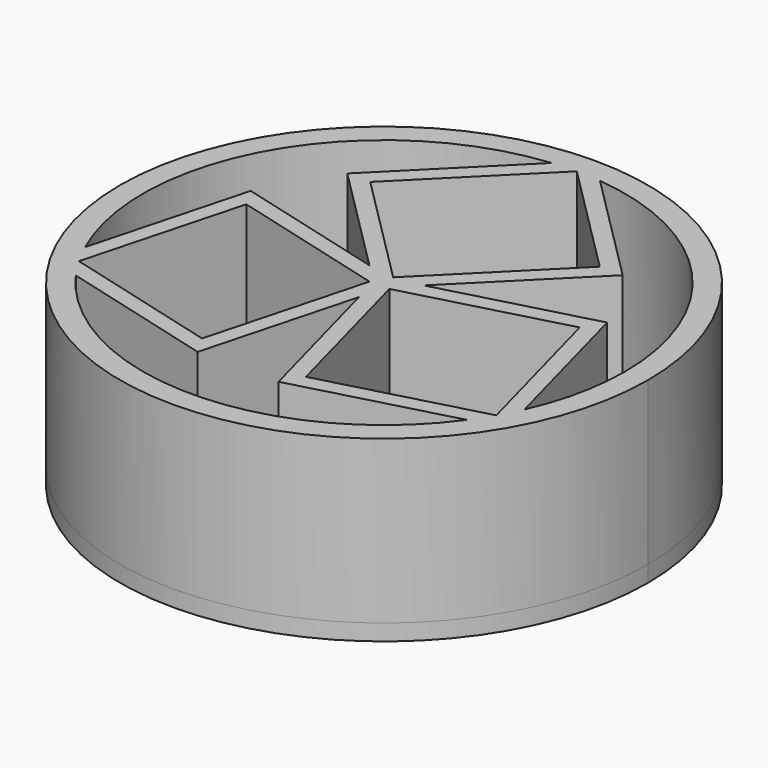
from build123d import *
from build123d import SkipClean  # not in build123d's __all__

# Parameters (mm, degrees)
F1_DEPTH = 1
F2_DEPTH = 10


with BuildPart() as f1:
    # F0 (on Top) → F1 (new body)
    with BuildSketch(Plane.XY):
        with BuildLine():
            Line((10.9787374798, 3.4593819318), (1.6730326075, 0.9659258263))
            Line((1.6730326075, 0.9659258263), (0.4482877361, -0.2588190451))
            Line((0.4482877361, -0.2588190451), (0, -1.9318516526))
            Line((0, -1.9318516526), (2.4934561055, -11.2375565249))
            Line((2.4934561055, -11.2375565249), (12.0504683321, -8.6767628167))
            ThreePointArc((12.0504683321, -8.6767628167), (12.4708698642, -8.0608563335), (12.8598211496, -7.4246212025))
            ThreePointArc((12.8598211496, -7.4246212025), (13.2163412932, -6.769661943), (13.5395311879, -6.0976302947))
            Line((13.5395311879, -6.0976302947), (10.9787374798, 3.4593819318))
        make_face()
        Polygon((10.2716306986, 2.2346370604), (12.8598211496, -7.4246212025), (3.2005628867, -10.0128116535), (0.6123724357, -0.3535533906), align=None, mode=Mode.SUBTRACT)
        with BuildLine():
            ThreePointArc((1.4890628559, 14.7743931114), (0.7454714289, 14.8305182765), (0, 14.8492424049))
            ThreePointArc((0, 14.8492424049), (-0.7454714289, 14.8305182765), (-1.4890628559, 14.7743931114))
            Line((-1.4890628559, 14.7743931114), (-8.4852813742, 7.7781745931))
            Line((-8.4852813742, 7.7781745931), (-1.6730326075, 0.9659258263))
            Line((-1.6730326075, 0.9659258263), (0, 0.5176380902))
            Line((0, 0.5176380902), (1.6730326075, 0.9659258263))
            Line((1.6730326075, 0.9659258263), (8.4852813742, 7.7781745931))
            Line((8.4852813742, 7.7781745931), (1.4890628559, 14.7743931114))
        make_face()
        Polygon((-7.0710678119, 7.7781745931), (0, 14.8492424049), (7.0710678119, 7.7781745931), (0, 0.7071067812), align=None, mode=Mode.SUBTRACT)
        with BuildLine():
            Line((-10.9787374798, 3.4593819318), (-13.5395311879, -6.0976302947))
            ThreePointArc((-13.5395311879, -6.0976302947), (-13.2163412932, -6.769661943), (-12.8598211496, -7.4246212025))
            ThreePointArc((-12.8598211496, -7.4246212025), (-12.4708698642, -8.0608563335), (-12.0504683321, -8.6767628167))
            Line((-12.0504683321, -8.6767628167), (-2.4934561055, -11.2375565249))
            Line((-2.4934561055, -11.2375565249), (0, -1.9318516526))
            Line((0, -1.9318516526), (-0.4482877361, -0.2588190451))
            Line((-0.4482877361, -0.2588190451), (-1.6730326075, 0.9659258263))
            Line((-1.6730326075, 0.9659258263), (-10.9787374798, 3.4593819318))
        make_face()
        Polygon((-3.2005628867, -10.0128116535), (-12.8598211496, -7.4246212025), (-10.2716306986, 2.2346370604), (-0.6123724357, -0.3535533906), align=None, mode=Mode.SUBTRACT)
        Polygon((-10.2716306986, 2.2346370604), (-12.8598211496, -7.4246212025), (-3.2005628867, -10.0128116535), (-0.6123724357, -0.3535533906), align=None)
        Polygon((3.2005628867, -10.0128116535), (12.8598211496, -7.4246212025), (10.2716306986, 2.2346370604), (0.6123724357, -0.3535533906), align=None)
        Polygon((7.0710678119, 7.7781745931), (0, 14.8492424049), (-7.0710678119, 7.7781745931), (0, 0.7071067812), align=None)
        with BuildLine():
            Line((-8.4852813742, 7.7781745931), (-1.4890628559, 14.7743931114))
            ThreePointArc((-1.4890628559, 14.7743931114), (-12.8598211496, 7.4246212025), (-13.5395311879, -6.0976302947))
            Line((-13.5395311879, -6.0976302947), (-10.9787374798, 3.4593819318))
            Line((-10.9787374798, 3.4593819318), (-1.6730326075, 0.9659258263))
            Line((-1.6730326075, 0.9659258263), (-8.4852813742, 7.7781745931))
        make_face()
        with BuildLine():
            ThreePointArc((14.8492424049, 0), (11.0138879444, 9.9596321392), (1.4890628559, 14.7743931114))
            Line((1.4890628559, 14.7743931114), (8.4852813742, 7.7781745931))
            Line((8.4852813742, 7.7781745931), (1.6730326075, 0.9659258263))
            Line((1.6730326075, 0.9659258263), (10.9787374798, 3.4593819318))
            Line((10.9787374798, 3.4593819318), (13.5395311879, -6.0976302947))
            ThreePointArc((13.5395311879, -6.0976302947), (14.5181228239, -3.1183504727), (14.8492424049, 0))
        make_face()
        with BuildLine():
            Line((-2.4934561055, -11.2375565249), (-12.0504683321, -8.6767628167))
            ThreePointArc((-12.0504683321, -8.6767628167), (0, -14.8492424049), (12.0504683321, -8.6767628167))
            Line((12.0504683321, -8.6767628167), (2.4934561055, -11.2375565249))
            Line((2.4934561055, -11.2375565249), (0, -1.9318516526))
            Line((0, -1.9318516526), (-2.4934561055, -11.2375565249))
        make_face()
        with BuildLine():
            ThreePointArc((-13.5395311879, -6.0976302947), (-12.8598211496, 7.4246212025), (-1.4890628559, 14.7743931114))
            Line((-1.4890628559, 14.7743931114), (0, 16.2634559673))
            ThreePointArc((0, 16.2634559673), (-14.084566021, 8.1317279836), (-14.084566021, -8.1317279836))
            Line((-14.084566021, -8.1317279836), (-13.5395311879, -6.0976302947))
        make_face()
        with BuildLine():
            Line((0, 16.2634559673), (1.4890628559, 14.7743931114))
            ThreePointArc((1.4890628559, 14.7743931114), (11.0138879444, 9.9596321392), (14.8492424049, 0))
            ThreePointArc((14.8492424049, 0), (14.5181228239, -3.1183504727), (13.5395311879, -6.0976302947))
            Line((13.5395311879, -6.0976302947), (14.084566021, -8.1317279836))
            ThreePointArc((14.084566021, -8.1317279836), (15.7092921435, -4.2092921435), (16.2634559673, 0))
            ThreePointArc((16.2634559673, 0), (11.5, 11.5), (0, 16.2634559673))
        make_face()
        with BuildLine():
            Line((-12.0504683321, -8.6767628167), (-14.084566021, -8.1317279836))
            ThreePointArc((-14.084566021, -8.1317279836), (0, -16.2634559673), (14.084566021, -8.1317279836))
            Line((14.084566021, -8.1317279836), (12.0504683321, -8.6767628167))
            ThreePointArc((12.0504683321, -8.6767628167), (0, -14.8492424049), (-12.0504683321, -8.6767628167))
        make_face()
        with BuildLine():
            ThreePointArc((-1.4890628559, 14.7743931114), (-0.7454714289, 14.8305182765), (0, 14.8492424049))
            ThreePointArc((0, 14.8492424049), (0.7454714289, 14.8305182765), (1.4890628559, 14.7743931114))
            Line((1.4890628559, 14.7743931114), (0, 16.2634559673))
            Line((0, 16.2634559673), (-1.4890628559, 14.7743931114))
        make_face()
        with BuildLine():
            Line((14.084566021, -8.1317279836), (13.5395311879, -6.0976302947))
            ThreePointArc((13.5395311879, -6.0976302947), (13.2163412932, -6.769661943), (12.8598211496, -7.4246212025))
            ThreePointArc((12.8598211496, -7.4246212025), (12.4708698642, -8.0608563335), (12.0504683321, -8.6767628167))
            Line((12.0504683321, -8.6767628167), (14.084566021, -8.1317279836))
        make_face()
        with BuildLine():
            ThreePointArc((-12.8598211496, -7.4246212025), (-13.2163412932, -6.769661943), (-13.5395311879, -6.0976302947))
            Line((-13.5395311879, -6.0976302947), (-14.084566021, -8.1317279836))
            Line((-14.084566021, -8.1317279836), (-12.0504683321, -8.6767628167))
            ThreePointArc((-12.0504683321, -8.6767628167), (-12.4708698642, -8.0608563335), (-12.8598211496, -7.4246212025))
        make_face()
        Polygon((0, -0.7071067812), (0.4482877361, -0.2588190451), (0.6123724357, 0.3535533906), (0, 0.5176380902), (-0.6123724357, 0.3535533906), (-0.4482877361, -0.2588190451), align=None)
        Polygon((0, -1.9318516526), (0.4482877361, -0.2588190451), (0, -0.7071067812), (-0.4482877361, -0.2588190451), align=None)
        Polygon((0, 0.5176380902), (-1.6730326075, 0.9659258263), (-0.4482877361, -0.2588190451), (-0.6123724357, 0.3535533906), align=None)
        Polygon((0.4482877361, -0.2588190451), (1.6730326075, 0.9659258263), (0, 0.5176380902), (0.6123724357, 0.3535533906), align=None)
    extrude(amount=-F1_DEPTH)

    # F0 (on Top) → F2 (join)
    with BuildSketch(Plane.XY):
        with BuildLine():
            Line((10.9787374798, 3.4593819318), (1.6730326075, 0.9659258263))
            Line((1.6730326075, 0.9659258263), (0.4482877361, -0.2588190451))
            Line((0.4482877361, -0.2588190451), (0, -1.9318516526))
            Line((0, -1.9318516526), (2.4934561055, -11.2375565249))
            Line((2.4934561055, -11.2375565249), (12.0504683321, -8.6767628167))
            ThreePointArc((12.0504683321, -8.6767628167), (12.4708698642, -8.0608563335), (12.8598211496, -7.4246212025))
            ThreePointArc((12.8598211496, -7.4246212025), (13.2163412932, -6.769661943), (13.5395311879, -6.0976302947))
            Line((13.5395311879, -6.0976302947), (10.9787374798, 3.4593819318))
        make_face()
        Polygon((10.2716306986, 2.2346370604), (12.8598211496, -7.4246212025), (3.2005628867, -10.0128116535), (0.6123724357, -0.3535533906), align=None, mode=Mode.SUBTRACT)
        with BuildLine():
            Line((0, 16.2634559673), (1.4890628559, 14.7743931114))
            ThreePointArc((1.4890628559, 14.7743931114), (11.0138879444, 9.9596321392), (14.8492424049, 0))
            ThreePointArc((14.8492424049, 0), (14.5181228239, -3.1183504727), (13.5395311879, -6.0976302947))
            Line((13.5395311879, -6.0976302947), (14.084566021, -8.1317279836))
            ThreePointArc((14.084566021, -8.1317279836), (15.7092921435, -4.2092921435), (16.2634559673, 0))
            ThreePointArc((16.2634559673, 0), (11.5, 11.5), (0, 16.2634559673))
        make_face()
        with BuildLine():
            ThreePointArc((-13.5395311879, -6.0976302947), (-12.8598211496, 7.4246212025), (-1.4890628559, 14.7743931114))
            Line((-1.4890628559, 14.7743931114), (0, 16.2634559673))
            ThreePointArc((0, 16.2634559673), (-14.084566021, 8.1317279836), (-14.084566021, -8.1317279836))
            Line((-14.084566021, -8.1317279836), (-13.5395311879, -6.0976302947))
        make_face()
        with BuildLine():
            ThreePointArc((1.4890628559, 14.7743931114), (0.7454714289, 14.8305182765), (0, 14.8492424049))
            ThreePointArc((0, 14.8492424049), (-0.7454714289, 14.8305182765), (-1.4890628559, 14.7743931114))
            Line((-1.4890628559, 14.7743931114), (-8.4852813742, 7.7781745931))
            Line((-8.4852813742, 7.7781745931), (-1.6730326075, 0.9659258263))
            Line((-1.6730326075, 0.9659258263), (0, 0.5176380902))
            Line((0, 0.5176380902), (1.6730326075, 0.9659258263))
            Line((1.6730326075, 0.9659258263), (8.4852813742, 7.7781745931))
            Line((8.4852813742, 7.7781745931), (1.4890628559, 14.7743931114))
        make_face()
        Polygon((-7.0710678119, 7.7781745931), (0, 14.8492424049), (7.0710678119, 7.7781745931), (0, 0.7071067812), align=None, mode=Mode.SUBTRACT)
        with BuildLine():
            Line((-12.0504683321, -8.6767628167), (-14.084566021, -8.1317279836))
            ThreePointArc((-14.084566021, -8.1317279836), (0, -16.2634559673), (14.084566021, -8.1317279836))
            Line((14.084566021, -8.1317279836), (12.0504683321, -8.6767628167))
            ThreePointArc((12.0504683321, -8.6767628167), (0, -14.8492424049), (-12.0504683321, -8.6767628167))
        make_face()
        with BuildLine():
            Line((-10.9787374798, 3.4593819318), (-13.5395311879, -6.0976302947))
            ThreePointArc((-13.5395311879, -6.0976302947), (-13.2163412932, -6.769661943), (-12.8598211496, -7.4246212025))
            ThreePointArc((-12.8598211496, -7.4246212025), (-12.4708698642, -8.0608563335), (-12.0504683321, -8.6767628167))
            Line((-12.0504683321, -8.6767628167), (-2.4934561055, -11.2375565249))
            Line((-2.4934561055, -11.2375565249), (0, -1.9318516526))
            Line((0, -1.9318516526), (-0.4482877361, -0.2588190451))
            Line((-0.4482877361, -0.2588190451), (-1.6730326075, 0.9659258263))
            Line((-1.6730326075, 0.9659258263), (-10.9787374798, 3.4593819318))
        make_face()
        Polygon((-3.2005628867, -10.0128116535), (-12.8598211496, -7.4246212025), (-10.2716306986, 2.2346370604), (-0.6123724357, -0.3535533906), align=None, mode=Mode.SUBTRACT)
        Polygon((0, -1.9318516526), (0.4482877361, -0.2588190451), (0, -0.7071067812), (-0.4482877361, -0.2588190451), align=None)
        with BuildLine():
            ThreePointArc((-1.4890628559, 14.7743931114), (-0.7454714289, 14.8305182765), (0, 14.8492424049))
            ThreePointArc((0, 14.8492424049), (0.7454714289, 14.8305182765), (1.4890628559, 14.7743931114))
            Line((1.4890628559, 14.7743931114), (0, 16.2634559673))
            Line((0, 16.2634559673), (-1.4890628559, 14.7743931114))
        make_face()
        Polygon((0, 0.5176380902), (-1.6730326075, 0.9659258263), (-0.4482877361, -0.2588190451), (-0.6123724357, 0.3535533906), align=None)
        with BuildLine():
            ThreePointArc((-12.8598211496, -7.4246212025), (-13.2163412932, -6.769661943), (-13.5395311879, -6.0976302947))
            Line((-13.5395311879, -6.0976302947), (-14.084566021, -8.1317279836))
            Line((-14.084566021, -8.1317279836), (-12.0504683321, -8.6767628167))
            ThreePointArc((-12.0504683321, -8.6767628167), (-12.4708698642, -8.0608563335), (-12.8598211496, -7.4246212025))
        make_face()
        with BuildLine():
            Line((14.084566021, -8.1317279836), (13.5395311879, -6.0976302947))
            ThreePointArc((13.5395311879, -6.0976302947), (13.2163412932, -6.769661943), (12.8598211496, -7.4246212025))
            ThreePointArc((12.8598211496, -7.4246212025), (12.4708698642, -8.0608563335), (12.0504683321, -8.6767628167))
            Line((12.0504683321, -8.6767628167), (14.084566021, -8.1317279836))
        make_face()
        Polygon((0.4482877361, -0.2588190451), (1.6730326075, 0.9659258263), (0, 0.5176380902), (0.6123724357, 0.3535533906), align=None)
        Polygon((0, -0.7071067812), (0.4482877361, -0.2588190451), (0.6123724357, 0.3535533906), (0, 0.5176380902), (-0.6123724357, 0.3535533906), (-0.4482877361, -0.2588190451), align=None)
    with SkipClean():  # cleaning this boolean's faces spoils the solid; the shape is the same uncleaned
        extrude(amount=F2_DEPTH)


solid = f1.part
